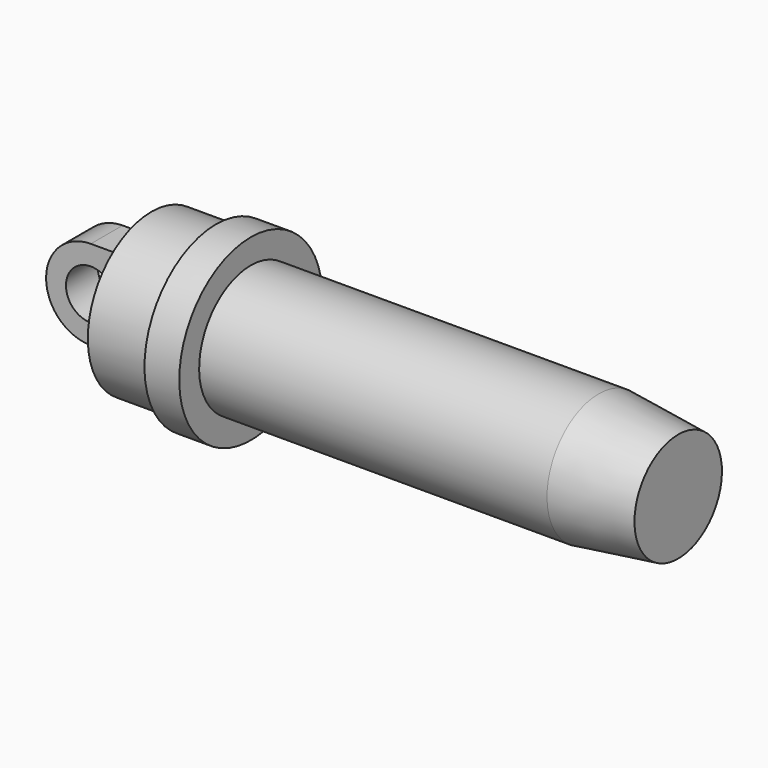
from build123d import *

# Parameters (mm, degrees)
F0_R     = 2.5
F1_DEPTH = 2


# Not quite as in the source:
# - a feature names something its author has since deleted; it is built from what else it names


with BuildPart() as f1:
    # F0 (on Front) → F1 (new body, symmetric)
    with BuildSketch(Plane.XZ):
        with BuildLine():
            Line((4.5, 4.5), (0, 4.5))
            ThreePointArc((0, 4.5), (-4.5, 0), (0, -4.5))
            Line((0, -4.5), (4.5, -4.5))
            Line((4.5, -4.5), (4.5, 0))
            Line((4.5, 0), (4.5, 4.5))
        make_face()
        Circle(F0_R, mode=Mode.SUBTRACT)
    extrude(amount=F1_DEPTH, both=True)

    # F0 (on Front) → F2 (revolve)
    with BuildSketch(Plane.XZ):
        Polygon((4.5, 8), (4.5, 4.5), (4.5, 0), (57.5, 0), (57.5, 5.5), (49.5, 6.5), (14.5, 6.5), (14.5, 9), (11, 9), (11, 8), align=None)
    revolve(axis=Axis((31, 0, 0), (1, 0, 0)))


solid = f1.part
